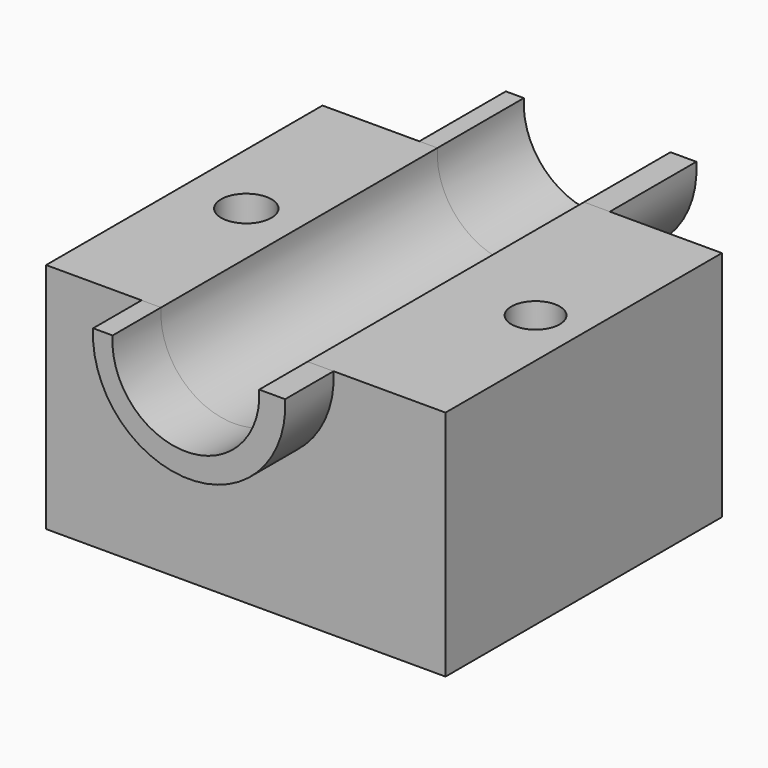
from build123d import *
from build123d import SkipClean  # not in build123d's __all__

# Parameters (mm, degrees)
F0_W     = 93.8486419618
F0_H     = 81.169269979
F1_DEPTH = 54.61
F3_DEPTH = 106.426
F4_DEPTH = 14.224
F6_DEPTH = 25.4
F7_R     = 5.6825549867
F7_R_2   = 5.9178586753
F8_DEPTH = 85.598


# Not quite as in the source:
# - after a boolean that leaves OpenCascade's solid faulty, fix() repairs it


with BuildPart() as f1:
    # F0 (on Top) → F1 (new body)
    with BuildSketch(Plane.XY):
        with Locations((-6.1729941517, 13.6784166098)):
            Rectangle(F0_W, F0_H)
    extrude(amount=F1_DEPTH)

    # F2 (on face) → F3 (cut)
    with BuildSketch(Plane.XZ.offset(26.9062183797)):
        with BuildLine():
            Line((8.3481688052, 54.61), (-26.0948427022, 54.61))
            ThreePointArc((-26.0948427022, 54.61), (-8.8733369485, 36.1893553029), (8.3481688052, 54.61))
        make_face()
    extrude(amount=-F3_DEPTH, mode=Mode.SUBTRACT)

    # F2 (on face) → F4 (join)
    with BuildSketch(Plane.XZ.offset(26.9062183797)):
        with BuildLine():
            Line((-26.0948427022, 54.61), (-30.6669250131, 54.61))
            ThreePointArc((-30.6669250131, 54.61), (-8.1113255583, 30.7368959369), (14.4442738965, 54.61))
            Line((14.4442738965, 54.61), (8.3481688052, 54.61))
            ThreePointArc((8.3481688052, 54.61), (-8.8733369485, 36.1893553029), (-26.0948427022, 54.61))
        make_face()
    with SkipClean():  # cleaning this boolean's faces spoils the solid; the shape is the same uncleaned
        extrude(amount=F4_DEPTH)

    # F5 (on face) → F6 (join)
    with BuildSketch(Plane(origin=(0, 54.2630515993, 0), x_dir=(-1, 0, 0), z_dir=(0, 1, 0))):
        with BuildLine():
            Line((-8.3481688052, 54.61), (-14.4147723913, 54.61))
            ThreePointArc((-14.4147723913, 54.61), (7.9621765763, 30.6739396567), (30.3391255438, 54.61))
            Line((30.3391255438, 54.61), (26.0948427022, 54.61))
            ThreePointArc((26.0948427022, 54.61), (8.8733369485, 36.1893553029), (-8.3481688052, 54.61))
        make_face()
    extrude(amount=F6_DEPTH)

    add(f1.part.fix(), mode=Mode.REPLACE)

    # F7 (on face) → F8 (cut)
    with BuildSketch(Plane.XY.offset(54.61)):
        with Locations((29.5217633247, 13.5689973831)):
            Circle(F7_R)
        with Locations((-38.4385436773, 13.5689973831)):
            Circle(F7_R_2)
    extrude(amount=-F8_DEPTH, mode=Mode.SUBTRACT)


solid = f1.part
